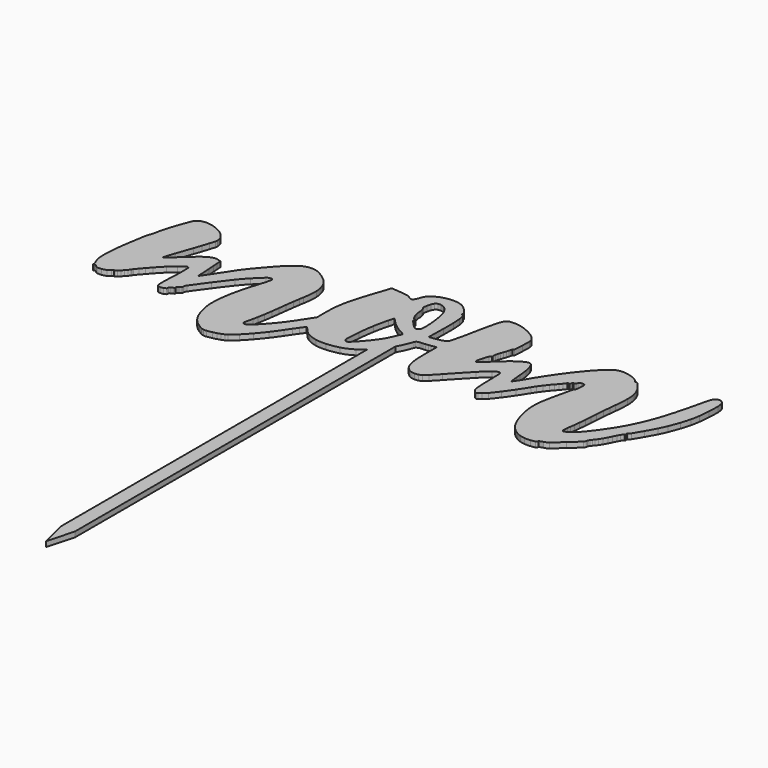
from build123d import *

# Parameters (mm, degrees)
F1_DEPTH = 1.5
F2_W     = 4
F2_H     = 115
F3_DEPTH = 1.5


# Not quite as in the source:
# - ends of sketch curves that miss each other by under 0.0002 mm in the source are joined


with BuildPart() as f1:
    # F0 (on Top) → F1 (new body)
    with BuildSketch(Plane.XY):
        with BuildLine():
            ThreePointArc((-4.1822559425, 22.5586507226), (-4.9915219103, 22.2917572117), (-5.7695987676, 21.9442806557))
            ThreePointArc((-5.7695987676, 21.9442806557), (-6.2638855218, 21.6755378797), (-6.742794415, 21.3802611645))
            ThreePointArc((-6.742794415, 21.3802611645), (-7.0841996448, 21.125395576), (-7.3917539608, 20.8305662103))
            ThreePointArc((-7.3917539608, 20.8305662103), (-7.6477142146, 20.5133884844), (-7.8596836812, 20.1652702398))
            ThreePointArc((-7.8596836812, 20.1652702398), (-8.0756822418, 19.7125223093), (-8.2587705459, 19.2454947615))
            ThreePointArc((-8.2587705459, 19.2454947615), (-8.4853451121, 18.6537844208), (-8.7444978395, 18.0756001689))
            ThreePointArc((-8.7444978395, 18.0756001689), (-8.9340338612, 17.8082033995), (-9.2009096557, 17.6179345962))
            ThreePointArc((-9.2009096557, 17.6179345962), (-9.4804778392, 17.5526269678), (-9.7609347332, 17.6140061624))
            ThreePointArc((-9.7609347332, 17.6140061624), (-10.1884309035, 17.8422128124), (-10.5897050006, 18.1138934121))
            ThreePointArc((-10.5897050006, 18.1138934121), (-10.9867832416, 18.3421223205), (-11.4282019209, 18.4642251951))
            ThreePointArc((-11.4282019209, 18.4642251951), (-12.5305443305, 18.6102904676), (-13.636129456, 18.7293508491))
            ThreePointArc((-13.636129456, 18.7293508491), (-14.7733093794, 18.8288693961), (-15.9118961479, 18.9107369284))
            ThreePointArc((-15.9118961479, 18.9107369284), (-16.1103487756, 18.8404745111), (-16.1965585813, 18.648411639))
            ThreePointArc((-16.1965585813, 18.648411639), (-16.200373914, 18.6073011501), (-16.210286377, 18.5672215402))
            ThreePointArc((-16.210286377, 18.5672215402), (-16.419979603, 17.9292142659), (-16.6298537231, 17.2912664743))
            ThreePointArc((-16.6298537231, 17.2912664743), (-16.8667329929, 16.574072426), (-17.1050936702, 15.8573693638))
            ThreePointArc((-17.1050936702, 15.8573693638), (-17.3865224907, 15.0158730838), (-17.6690280218, 14.1747376637))
            ThreePointArc((-17.6690280218, 14.1747376637), (-18.3536086298, 12.0776659538), (-18.9998070552, 9.9684509451))
            ThreePointArc((-18.9998070552, 9.9684509451), (-19.434349035, 8.3783522453), (-19.8004649353, 6.771118674))
            ThreePointArc((-19.8004649353, 6.771118674), (-20.0490192241, 5.3746056153), (-20.2234246645, 3.9669086683))
            ThreePointArc((-20.2234246645, 3.9669086683), (-20.3294158982, 2.5100215792), (-20.3647728593, 1.0497120123))
            Line((-20.3647728593, 1.0497120123), (-20.3647728593, -2.4233168496))
            Line((-20.3647728593, -2.4233168496), (-22.919139759, -6.3134028131))
            ThreePointArc((-22.919139759, -6.3134028131), (-23.9837763775, -7.8648103517), (-25.110819257, -9.3714924057))
            ThreePointArc((-25.110819257, -9.3714924057), (-26.2997155674, -10.8327814282), (-27.5470323246, -12.2445324531))
            ThreePointArc((-27.5470323246, -12.2445324531), (-28.6699490161, -13.4282570975), (-29.8280346413, -14.5775976193))
            ThreePointArc((-29.8280346413, -14.5775976193), (-30.3391428464, -14.9087464889), (-30.9370028544, -15.0247401796))
            ThreePointArc((-30.9370028544, -15.0247401796), (-31.1663651817, -14.9984768587), (-31.3838541049, -14.9210468419))
            ThreePointArc((-31.3838541049, -14.9210468419), (-31.5089949751, -14.808872531), (-31.5571193403, -14.6478527512))
            ThreePointArc((-31.5571193403, -14.6478527512), (-31.5428967438, -14.3333788672), (-31.4906101134, -14.0229562465))
            ThreePointArc((-31.4906101134, -14.0229562465), (-31.2411328819, -12.9594000391), (-30.985931045, -11.8972029212))
            ThreePointArc((-30.985931045, -11.8972029212), (-30.8380868978, -11.2453452123), (-30.7104532496, -10.5892308852))
            ThreePointArc((-30.7104532496, -10.5892308852), (-30.5374868635, -9.5932928505), (-30.3739315542, -8.5957661091))
            ThreePointArc((-30.3739315542, -8.5957661091), (-30.2012078519, -7.4762107698), (-30.0390624167, -6.3550745191))
            ThreePointArc((-30.0390624167, -6.3550745191), (-29.8922592615, -5.2641425918), (-29.7566894255, -4.1717578345))
            ThreePointArc((-29.7566894255, -4.1717578345), (-29.6251269486, -3.0895293391), (-29.4878411294, -2.0080119761))
            ThreePointArc((-29.4878411294, -2.0080119761), (-29.3435223079, -0.916672936), (-29.1935983974, 0.17391023))
            ThreePointArc((-29.1935983974, 0.17391023), (-29.0568759692, 1.1321864661), (-28.9152986168, 2.0897574667))
            ThreePointArc((-28.9152986168, 2.0897574667), (-28.8192464519, 2.6893466621), (-28.7117907934, 3.2869974804))
            ThreePointArc((-28.7117907934, 3.2869974804), (-28.4328255875, 5.2872447136), (-28.3503002579, 7.3051644583))
            ThreePointArc((-28.3503002579, 7.3051644583), (-28.5212434867, 8.8744231228), (-29.0021338886, 10.37793196))
            ThreePointArc((-29.0021338886, 10.37793196), (-29.7451965352, 11.6773360862), (-30.7525232215, 12.7845334956))
            ThreePointArc((-30.7525232215, 12.7845334956), (-32.16418877, 13.8757158075), (-33.7057215553, 14.7741339442))
            ThreePointArc((-33.7057215553, 14.7741339442), (-34.9524958644, 15.2120375761), (-36.2687880295, 15.3285737489))
            ThreePointArc((-36.2687880295, 15.3285737489), (-37.5645264585, 15.1148542043), (-38.764947663, 14.5823103026))
            ThreePointArc((-38.764947663, 14.5823103026), (-40.3221476085, 13.4878304003), (-41.7164387191, 12.1921799081))
            ThreePointArc((-41.7164387191, 12.1921799081), (-43.9120092144, 9.7823205671), (-46.0338372664, 7.3072857043))
            ThreePointArc((-46.0338372664, 7.3072857043), (-46.4456634194, 6.8082415191), (-46.8538054567, 6.3061798129))
            ThreePointArc((-46.8538054567, 6.3061798129), (-47.235224243, 5.8291917787), (-47.612454984, 5.3488847494))
            ThreePointArc((-47.612454984, 5.3488847494), (-47.9271786213, 4.9413426126), (-48.2387883176, 4.5314146198))
            ThreePointArc((-48.2387883176, 4.5314146198), (-48.3814207795, 4.3308497903), (-48.5126087033, 4.1226191562))
            ThreePointArc((-48.5126087033, 4.1226191562), (-48.6473158751, 3.9001325822), (-48.7865416946, 3.6804453742))
            ThreePointArc((-48.7865416946, 3.6804453742), (-49.1331745219, 3.1467861518), (-49.4808420237, 2.6138004196))
            ThreePointArc((-49.4808420237, 2.6138004196), (-49.8968100308, 1.9791749235), (-50.3143492141, 1.3455820469))
            ThreePointArc((-50.3143492141, 1.3455820469), (-50.7680770752, 0.6603827725), (-51.2231413323, -0.0239296847))
            Line((-51.2231413323, -0.0239296847), (-53.5166684536, -3.4655815887))
            Line((-53.5166684536, -3.4655815887), (-53.7783240639, 0.8672097846))
            ThreePointArc((-53.7783240639, 0.8672097846), (-53.8294707555, 1.6999810285), (-53.8823208533, 2.5326459042))
            ThreePointArc((-53.8823208533, 2.5326459042), (-53.9290447639, 3.2386970453), (-53.9781283051, 3.944588074))
            ThreePointArc((-53.9781283051, 3.944588074), (-54.0230894341, 4.5743024761), (-54.0682833336, 5.2040002153))
            ThreePointArc((-54.0682833336, 5.2040002153), (-54.0752279531, 5.2333667956), (-54.0910777713, 5.2590457477))
            ThreePointArc((-54.0910777713, 5.2590457477), (-54.1122644757, 5.2775060716), (-54.1377439385, 5.2893575669))
            ThreePointArc((-54.1377439385, 5.2893575669), (-54.2859965399, 5.3339698764), (-54.434460934, 5.3778722185))
            ThreePointArc((-54.434460934, 5.3778722185), (-54.6087752013, 5.4278455529), (-54.7836692699, 5.4757502762))
            ThreePointArc((-54.7836692699, 5.4757502762), (-54.9857744892, 5.5289837999), (-55.1882867028, 5.5806474337))
            ThreePointArc((-55.1882867028, 5.5806474337), (-55.7750569441, 5.6525847428), (-56.3615460507, 5.5783902643))
            ThreePointArc((-56.3615460507, 5.5783902643), (-57.0397471351, 5.3530815554), (-57.6792417151, 5.0340715138))
            ThreePointArc((-57.6792417151, 5.0340715138), (-58.5489239003, 4.4695325207), (-59.3681127786, 3.8339375469))
            ThreePointArc((-59.3681127786, 3.8339375469), (-60.6078625294, 2.7611061181), (-61.8227559636, 1.6602061928))
            ThreePointArc((-61.8227559636, 1.6602061928), (-62.4322452312, 1.0981496578), (-63.0447760209, 0.5394093375))
            ThreePointArc((-63.0447760209, 0.5394093375), (-63.5721918871, 0.0650609012), (-64.1036845799, -0.4047150597))
            ThreePointArc((-64.1036845799, -0.4047150597), (-64.5687800812, -0.81133911), (-65.0347655754, -1.2169429345))
            ThreePointArc((-65.0347655754, -1.2169429345), (-65.0929570576, -1.2515369423), (-65.1595758219, -1.2635759706))
            ThreePointArc((-65.1595758219, -1.2635759706), (-65.2465892772, -1.2202875127), (-65.264550455, -1.1247750628))
            ThreePointArc((-65.264550455, -1.1247750628), (-65.1010382295, -0.5630542496), (-64.9291088642, -0.0038523054))
            ThreePointArc((-64.9291088642, -0.0038523054), (-64.6191741236, 0.9558542093), (-64.2966272322, 1.9113957541))
            ThreePointArc((-64.2966272322, 1.9113957541), (-63.5118912001, 4.1817279915), (-62.7241409714, 6.4510161364))
            ThreePointArc((-62.7241409714, 6.4510161364), (-62.3584274565, 7.5153052648), (-62.0008194789, 8.5823452167))
            ThreePointArc((-62.0008194789, 8.5823452167), (-61.6896775555, 9.5395945184), (-61.3887147953, 10.5000927935))
            ThreePointArc((-61.3887147953, 10.5000927935), (-61.1430588832, 11.308414842), (-60.9027515407, 12.1183430759))
            ThreePointArc((-60.9027515407, 12.1183430759), (-60.8475182031, 12.3678683627), (-60.826260255, 12.6225479491))
            ThreePointArc((-60.826260255, 12.6225479491), (-60.8760261629, 13.2132637936), (-61.0422047693, 13.7823037851))
            ThreePointArc((-61.0422047693, 13.7823037851), (-61.3327877583, 14.3721380824), (-61.7067140299, 14.9129912493))
            ThreePointArc((-61.7067140299, 14.9129912493), (-62.2131221431, 15.4658692638), (-62.7850651647, 15.950641847))
            ThreePointArc((-62.7850651647, 15.950641847), (-63.4832237539, 16.4237718816), (-64.2206136701, 16.8330804933))
            ThreePointArc((-64.2206136701, 16.8330804933), (-65.1252901816, 17.2383089572), (-66.0602335864, 17.5677486859))
            ThreePointArc((-66.0602335864, 17.5677486859), (-66.9070821685, 17.7724206835), (-67.7724364315, 17.8734411577))
            ThreePointArc((-67.7724364315, 17.8734411577), (-68.5155243267, 17.8609951412), (-69.2490163874, 17.7413126029))
            ThreePointArc((-69.2490163874, 17.7413126029), (-69.853154693, 17.5236256148), (-70.3941183825, 17.1776067625))
            ThreePointArc((-70.3941183825, 17.1776067625), (-70.8092834506, 16.7433928091), (-71.1018494221, 16.2186938699))
            ThreePointArc((-71.1018494221, 16.2186938699), (-71.6814891859, 14.7304548726), (-72.231005615, 13.2308318357))
            ThreePointArc((-72.231005615, 13.2308318357), (-72.7813626503, 11.6050767122), (-73.2835471725, 9.9638018107))
            ThreePointArc((-73.2835471725, 9.9638018107), (-73.664727082, 8.5280649184), (-73.9804265564, 7.076523538))
            ThreePointArc((-73.9804265564, 7.076523538), (-74.0261796134, 6.8535167435), (-74.076771101, 6.6315575731))
            ThreePointArc((-74.076771101, 6.6315575731), (-74.135954279, 6.3934993523), (-74.1992682126, 6.1565062898))
            ThreePointArc((-74.1992682126, 6.1565062898), (-74.2617462221, 5.9380485217), (-74.328061585, 5.7207248687))
            ThreePointArc((-74.328061585, 5.7207248687), (-74.3814168207, 5.5633688503), (-74.4416203428, 5.4085036385))
            ThreePointArc((-74.4416203428, 5.4085036385), (-74.4994993237, 5.2601300671), (-74.5511683002, 5.1094814382))
            ThreePointArc((-74.5511683002, 5.1094814382), (-74.6108233058, 4.9162070008), (-74.6664979641, 4.7217486211))
            ThreePointArc((-74.6664979641, 4.7217486211), (-74.7202513052, 4.5183855512), (-74.7698584316, 4.3139715286))
            ThreePointArc((-74.7698584316, 4.3139715286), (-74.8092636056, 4.1320166537), (-74.8433256505, 3.9489862685))
            ThreePointArc((-74.8433256505, 3.9489862685), (-75.3714936754, 0.7359748324), (-75.8583007895, -2.4835628313))
            ThreePointArc((-75.8583007895, -2.4835628313), (-76.1231681958, -4.629163355), (-76.2985191984, -6.7839274669))
            ThreePointArc((-76.2985191984, -6.7839274669), (-76.3428147207, -8.2970233342), (-76.2929072344, -9.8099444977))
            ThreePointArc((-76.2929072344, -9.8099444977), (-76.1345866751, -10.8741643639), (-75.8013874655, -11.8972027673))
            ThreePointArc((-75.8013874655, -11.8972027673), (-75.6999104882, -12.1479333715), (-75.6054305509, -12.4013834739))
            ThreePointArc((-75.6054305509, -12.4013834739), (-75.5247349489, -12.6402342171), (-75.4522677026, -12.8817087512))
            ThreePointArc((-75.4522677026, -12.8817087512), (-75.398642255, -13.0842728713), (-75.3513736965, -13.2884139943))
            ThreePointArc((-75.3513736965, -13.2884139943), (-75.3408090463, -13.3902479231), (-75.3524233081, -13.4919674365))
            ThreePointArc((-75.3524233081, -13.4919674365), (-75.3578141372, -13.5473192244), (-75.3493302057, -13.6022819056))
            ThreePointArc((-75.3493302057, -13.6022819056), (-75.3274262122, -13.6398650775), (-75.2902116395, -13.6623896439))
            ThreePointArc((-75.2902116395, -13.6623896439), (-75.2345411787, -13.6700441916), (-75.1792530029, -13.6599936843))
            ThreePointArc((-75.1792530029, -13.6599936843), (-75.1035087165, -13.6286877996), (-75.0315710199, -13.589416625))
            ThreePointArc((-75.0315710199, -13.589416625), (-74.9487622667, -13.5495723993), (-74.8594618396, -13.5278862888))
            ThreePointArc((-74.8594618396, -13.5278862888), (-74.7657183984, -13.5246792034), (-74.6731732176, -13.5399601928))
            ThreePointArc((-74.6731732176, -13.5399601928), (-74.5832645797, -13.5736545995), (-74.5014379699, -13.6238869091))
            ThreePointArc((-74.5014379699, -13.6238869091), (-74.4296336563, -13.6893500971), (-74.3711213165, -13.7669232111))
            ThreePointArc((-74.3711213165, -13.7669232111), (-74.0943971868, -14.0492003461), (-73.7232801093, -14.1853206266))
            ThreePointArc((-73.7232801093, -14.1853206266), (-73.1081117024, -14.2256966538), (-72.4928310229, -14.1870696251))
            ThreePointArc((-72.4928310229, -14.1870696251), (-71.8377271814, -14.0622844651), (-71.2028465133, -13.8581792676))
            ThreePointArc((-71.2028465133, -13.8581792676), (-70.7333802299, -13.6070314156), (-70.3361908816, -13.252469085))
            ThreePointArc((-70.3361908816, -13.252469085), (-70.1864087009, -13.0866749815), (-70.0328775637, -12.9243463791))
            ThreePointArc((-70.0328775637, -12.9243463791), (-69.9437306254, -12.8430726196), (-69.8451341813, -12.7735647379))
            ThreePointArc((-69.8451341813, -12.7735647379), (-69.8105070702, -12.7730112819), (-69.7934259349, -12.8031374144))
            ThreePointArc((-69.7934259349, -12.8031374144), (-69.8028215767, -12.8733789518), (-69.827754287, -12.9397153005))
            ThreePointArc((-69.827754287, -12.9397153005), (-69.8245031219, -12.9853701203), (-69.7825618234, -13.0036965528))
            ThreePointArc((-69.7825618234, -13.0036965528), (-69.6947559153, -12.9801297562), (-69.6159866251, -12.9347350445))
            ThreePointArc((-69.6159866251, -12.9347350445), (-69.4087154408, -12.767215773), (-69.2106525463, -12.5889038654))
            ThreePointArc((-69.2106525463, -12.5889038654), (-68.9316613256, -12.3191357057), (-68.6575720048, -12.0443885362))
            ThreePointArc((-68.6575720048, -12.0443885362), (-68.3643476946, -11.7405929424), (-68.0757154403, -11.4324311665))
            ThreePointArc((-68.0757154403, -11.4324311665), (-67.8151289864, -11.1444754722), (-67.5601404874, -10.851551169))
            ThreePointArc((-67.5601404874, -10.851551169), (-67.3518605409, -10.6037065546), (-67.147453089, -10.3526585847))
            ThreePointArc((-67.147453089, -10.3526585847), (-67.0716457549, -10.2412100141), (-67.0141409908, -10.1193054142))
            ThreePointArc((-67.0141409908, -10.1193054142), (-66.9483485935, -9.9811894042), (-66.8608755299, -9.855677946))
            ThreePointArc((-66.8608755299, -9.855677946), (-66.4558544705, -9.3681557388), (-66.0483968957, -8.8826680599))
            ThreePointArc((-66.0483968957, -8.8826680599), (-65.5626572142, -8.3125097497), (-65.0713750069, -7.7471202124))
            ThreePointArc((-65.0713750069, -7.7471202124), (-64.5087102139, -7.1102408743), (-63.9417931494, -6.477143721))
            ThreePointArc((-63.9417931494, -6.477143721), (-62.8969404894, -5.3490949705), (-61.8220698579, -4.2496113755))
            ThreePointArc((-61.8220698579, -4.2496113755), (-60.9263888483, -3.4028181835), (-59.9880774003, -2.6035217377))
            ThreePointArc((-59.9880774003, -2.6035217377), (-59.262628442, -2.0479626884), (-58.5091525982, -1.5310524402))
            ThreePointArc((-58.5091525982, -1.5310524402), (-58.1616557398, -1.4262262904), (-57.8119768273, -1.5235258845))
            ThreePointArc((-57.8119768273, -1.5235258845), (-57.7137215941, -1.6246169813), (-57.6748883547, -1.7601363133))
            ThreePointArc((-57.6748883547, -1.7601363133), (-57.6538185631, -2.5029076798), (-57.6396808543, -3.2458433181))
            ThreePointArc((-57.6396808543, -3.2458433181), (-57.6360432054, -4.1307602045), (-57.6505451458, -5.0155657315))
            ThreePointArc((-57.6505451458, -5.0155657315), (-57.6846924586, -6.0447961381), (-57.7322697912, -7.07349321))
            ThreePointArc((-57.7322697912, -7.07349321), (-57.7944578959, -8.3689613454), (-57.8442692694, -9.6649643838))
            ThreePointArc((-57.8442692694, -9.6649643838), (-57.856867574, -10.4757670984), (-57.8401082345, -11.286494475))
            ThreePointArc((-57.8401082345, -11.286494475), (-57.807360429, -11.8159482663), (-57.7502999635, -12.3433360171))
            ThreePointArc((-57.7502999635, -12.3433360171), (-57.673204314, -12.5529847958), (-57.5136494411, -12.7093133269))
            ThreePointArc((-57.5136494411, -12.7093133269), (-57.2054591723, -12.8426456929), (-56.8719905685, -12.8821103557))
            ThreePointArc((-56.8719905685, -12.8821103557), (-56.4211425786, -12.8420036032), (-55.9785762085, -12.7470959978))
            ThreePointArc((-55.9785762085, -12.7470959978), (-55.6225780145, -12.6171325954), (-55.2909196385, -12.4337534234))
            ThreePointArc((-55.2909196385, -12.4337534234), (-55.1755300418, -12.2660820174), (-55.2095904797, -12.0654121401))
            ThreePointArc((-55.2095904797, -12.0654121401), (-55.2429992614, -11.9770427378), (-55.2408434003, -11.8825934375))
            ThreePointArc((-55.2408434003, -11.8825934375), (-55.2042535921, -11.7811978242), (-55.1425856263, -11.6927843572))
            ThreePointArc((-55.1425856263, -11.6927843572), (-55.0388849343, -11.5981176824), (-54.9198375465, -11.5236641951))
            ThreePointArc((-54.9198375465, -11.5236641951), (-54.7659971521, -11.4558390196), (-54.6058283114, -11.4047208545))
            ThreePointArc((-54.6058283114, -11.4047208545), (-54.4447093367, -11.3547072715), (-54.2887639942, -11.2903509784))
            ThreePointArc((-54.2887639942, -11.2903509784), (-54.167268058, -11.2214926632), (-54.058122806, -11.134371819))
            ThreePointArc((-54.058122806, -11.134371819), (-53.9924301765, -11.0560024408), (-53.9473415092, -10.9642184766))
            ThreePointArc((-53.9473415092, -10.9642184766), (-53.937987883, -10.8823035628), (-53.9647940919, -10.8043358161))
            ThreePointArc((-53.9647940919, -10.8043358161), (-53.9964262926, -10.7265964996), (-54.000804246, -10.6427822877))
            ThreePointArc((-54.000804246, -10.6427822877), (-53.978910261, -10.5513457426), (-53.935896193, -10.4677408564))
            ThreePointArc((-53.935896193, -10.4677408564), (-53.8631232474, -10.3789790757), (-53.7754141586, -10.30494073))
            ThreePointArc((-53.7754141586, -10.30494073), (-53.6630098407, -10.2362111231), (-53.5430990436, -10.1816227544))
            ThreePointArc((-53.5430990436, -10.1816227544), (-53.4154851319, -10.1256275996), (-53.2937010792, -10.0578824381))
            ThreePointArc((-53.2937010792, -10.0578824381), (-53.1838223253, -9.9814396197), (-53.0826675643, -9.8937779729))
            ThreePointArc((-53.0826675643, -9.8937779729), (-53.0050697908, -9.8093331136), (-52.9382242426, -9.7161450243))
            ThreePointArc((-52.9382242426, -9.7161450243), (-52.9031619045, -9.637914576), (-52.8911609896, -9.5530302369))
            ThreePointArc((-52.8911609896, -9.5530302369), (-52.8055751283, -9.0065852313), (-52.5570144162, -8.5124752676))
            ThreePointArc((-52.5570144162, -8.5124752676), (-50.9049322696, -6.2203896441), (-49.2387076685, -3.9385641684))
            ThreePointArc((-49.2387076685, -3.9385641684), (-47.620417887, -1.7722741308), (-45.9685796397, 0.368544584))
            ThreePointArc((-45.9685796397, 0.368544584), (-44.8534491069, 1.7140619809), (-43.6671281303, 2.9972516342))
            ThreePointArc((-43.6671281303, 2.9972516342), (-42.4301332189, 4.2308010058), (-41.1602271105, 5.4304421727))
            ThreePointArc((-41.1602271105, 5.4304421727), (-40.6342141081, 5.7522390789), (-40.0254736735, 5.8506163559))
            ThreePointArc((-40.0254736735, 5.8506163559), (-39.6468333598, 5.661340297), (-39.5427213099, 5.2510300767))
            ThreePointArc((-39.5427213099, 5.2510300767), (-39.8013508117, 4.0542865399), (-40.1358962279, 2.8765074091))
            ThreePointArc((-40.1358962279, 2.8765074091), (-41.025635013, -0.0511910088), (-41.8349245611, -3.0021406109))
            ThreePointArc((-41.8349245611, -3.0021406109), (-42.3726246239, -5.3408386427), (-42.7786081902, -7.7059617258))
            ThreePointArc((-42.7786081902, -7.7059617258), (-42.985017337, -9.6396450101), (-43.0531009585, -11.5831213836))
            ThreePointArc((-43.0531009585, -11.5831213836), (-42.9576359866, -13.2428668027), (-42.6746090087, -14.8810866201))
            ThreePointArc((-42.6746090087, -14.8810866201), (-42.3511388295, -16.1104284713), (-41.9559710395, -17.3186324001))
            ThreePointArc((-41.9559710395, -17.3186324001), (-41.5479934206, -18.2935342997), (-41.0431893663, -19.2220020331))
            ThreePointArc((-41.0431893663, -19.2220020331), (-40.4997867922, -20.0043819358), (-39.8691379588, -20.7183053858))
            ThreePointArc((-39.8691379588, -20.7183053858), (-39.1527041487, -21.3630475184), (-38.3684380392, -21.9233121883))
            ThreePointArc((-38.3684380392, -21.9233121883), (-37.7803696665, -22.2807581428), (-37.1798687644, -22.6168990168))
            ThreePointArc((-37.1798687644, -22.6168990168), (-36.8187592337, -22.7726530636), (-36.4364715582, -22.8649328236))
            ThreePointArc((-36.4364715582, -22.8649328236), (-36.0255703165, -22.8960166594), (-35.6147111703, -22.8643813839))
            ThreePointArc((-35.6147111703, -22.8643813839), (-34.8322051067, -22.73353173), (-34.05326431, -22.5829043212))
            ThreePointArc((-34.05326431, -22.5829043212), (-33.5450667482, -22.4683826133), (-33.0413101397, -22.3356827592))
            ThreePointArc((-33.0413101397, -22.3356827592), (-32.5382415862, -22.1838969881), (-32.0407933742, -22.0145979308))
            ThreePointArc((-32.0407933742, -22.0145979308), (-31.6088795425, -21.8504218929), (-31.1830483815, -21.6710587133))
            ThreePointArc((-31.1830483815, -21.6710587133), (-30.9156435461, -21.5330041438), (-30.6667650025, -21.3638182089))
            ThreePointArc((-30.6667650025, -21.3638182089), (-29.6790688612, -20.5493797605), (-28.7459929373, -19.6728964566))
            ThreePointArc((-28.7459929373, -19.6728964566), (-27.6334299799, -18.520275589), (-26.5598745739, -17.3312381615))
            ThreePointArc((-26.5598745739, -17.3312381615), (-25.4284265627, -15.9933166985), (-24.3397287735, -14.620383499))
            ThreePointArc((-24.3397287735, -14.620383499), (-23.2970435644, -13.2164689104), (-22.2994122978, -11.7801888303))
            ThreePointArc((-22.2994122978, -11.7801888303), (-21.7461323637, -10.9615839169), (-21.1877421009, -10.1464563169))
            ThreePointArc((-21.1877421009, -10.1464563169), (-20.7064388551, -9.4560230246), (-20.2181990799, -8.7704773517))
            ThreePointArc((-20.2181990799, -8.7704773517), (-19.7895503223, -8.1765157547), (-19.3594479355, -7.5836059198))
            ThreePointArc((-19.3594479355, -7.5836059198), (-19.3034623423, -7.5358243614), (-19.2318904369, -7.5186506111))
            ThreePointArc((-19.2318904369, -7.5186506111), (-19.1686419514, -7.5305800964), (-19.1140845066, -7.5647293093))
            ThreePointArc((-19.1140845066, -7.5647293093), (-18.9770961812, -7.6943381598), (-18.8432663523, -7.8272058875))
            ThreePointArc((-18.8432663523, -7.8272058875), (-18.6841706893, -7.9943686056), (-18.5306061244, -8.1666263419))
            ThreePointArc((-18.5306061244, -8.1666263419), (-18.3625456012, -8.3659621524), (-18.199040705, -8.5690514311))
            ThreePointArc((-18.199040705, -8.5690514311), (-17.3531301887, -9.4416557191), (-16.3461412481, -10.12207919))
            ThreePointArc((-16.3461412481, -10.12207919), (-15.1159644234, -10.6628346337), (-13.8175853913, -11.0091919713))
            ThreePointArc((-13.8175853913, -11.0091919713), (-12.2858853212, -11.1921895086), (-10.7433888506, -11.1749306796))
            ThreePointArc((-10.7433888506, -11.1749306796), (-9.0034596895, -10.9638456428), (-7.2891719049, -10.5989788562))
            ThreePointArc((-7.2891719049, -10.5989788562), (-5.5072879501, -9.9724728868), (-3.8550637645, -9.0571721758))
            ThreePointArc((-3.8550637645, -9.0571721758), (-2.1773976949, -7.7809088725), (-0.6661841912, -6.3113357406))
            ThreePointArc((-0.6661841912, -6.3113357406), (0.780118398, -4.5348463442), (2.0206413229, -2.6090211129))
            ThreePointArc((2.0206413229, -2.6090211129), (3.101013261, -0.4720664298), (3.9687420637, 1.7597100373))
            ThreePointArc((3.9687420637, 1.7597100373), (4.0429607856, 1.9222699293), (4.1497565079, 2.0655487572))
            ThreePointArc((4.1497565079, 2.0655487572), (4.2918637926, 2.1949479823), (4.4539218623, 2.2982717748))
            ThreePointArc((4.4539218623, 2.2982717748), (4.6559590459, 2.3860996721), (4.8685089146, 2.444024833))
            ThreePointArc((4.8685089146, 2.444024833), (5.1191629671, 2.4810197731), (5.3721967094, 2.4940583415))
            ThreePointArc((5.3721967094, 2.4940583415), (5.6474109783, 2.4993711533), (5.9223326228, 2.513126545))
            ThreePointArc((5.9223326228, 2.513126545), (6.2759538804, 2.5388542458), (6.6291626887, 2.5697321278))
            ThreePointArc((6.6291626887, 2.5697321278), (6.9984444577, 2.6074183955), (7.3671439486, 2.6504296454))
            ThreePointArc((7.3671439486, 2.6504296454), (7.6953045038, 2.6945009672), (8.0225027057, 2.7452253932))
            Line((8.0225027057, 2.7452253932), (9.512956874, 2.9918030159))
            Line((9.512956874, 2.9918030159), (9.489490753, -1.1166601135))
            ThreePointArc((9.489490753, -1.1166601135), (9.5312740917, -3.2067309573), (9.6803820608, -5.2918949357))
            ThreePointArc((9.6803820608, -5.2918949357), (9.9288893063, -6.6590144491), (10.3991588685, -7.9665380884))
            ThreePointArc((10.3991588685, -7.9665380884), (10.9353106418, -8.8055932953), (11.6832726288, -9.4628795794))
            ThreePointArc((11.6832726288, -9.4628795794), (12.5765507142, -9.8782528649), (13.551330224, -10.0206804672))
            ThreePointArc((13.551330224, -10.0206804672), (14.0908782717, -9.9864098255), (14.6217540504, -9.8841480039))
            ThreePointArc((14.6217540504, -9.8841480039), (15.0692994731, -9.7226182531), (15.4794268286, -9.4814040321))
            ThreePointArc((15.4794268286, -9.4814040321), (16.0162580118, -9.0571422232), (16.5132514964, -8.5868409476))
            ThreePointArc((16.5132514964, -8.5868409476), (17.5599755317, -7.4925098038), (18.5950103109, -6.387116271))
            ThreePointArc((18.5950103109, -6.387116271), (21.1766435374, -3.6230930989), (23.7806788264, -0.8801650253))
            ThreePointArc((23.7806788264, -0.8801650253), (25.0803561969, 0.4005733241), (26.4526707118, 1.6031559035))
            ThreePointArc((26.4526707118, 1.6031559035), (27.0922293683, 2.0133090023), (27.8109979968, 2.2595457583))
            ThreePointArc((27.8109979968, 2.2595457583), (28.2507574872, 2.159610569), (28.4592161085, 1.7597101107))
            ThreePointArc((28.4592161085, 1.7597101107), (28.4692596352, 1.5208514025), (28.4768725053, 1.2819028765))
            ThreePointArc((28.4768725053, 1.2819028765), (28.4939603313, 0.6342572533), (28.5105505023, -0.0134013091))
            ThreePointArc((28.5105505023, -0.0134013091), (28.5296330893, -0.7859654794), (28.5478966907, -1.5585494446))
            ThreePointArc((28.5478966907, -1.5585494446), (28.5671175763, -2.405090089), (28.5856563176, -3.2516459466))
            ThreePointArc((28.5856563176, -3.2516459466), (28.6169098518, -4.3551611664), (28.6632158116, -5.4581472845))
            ThreePointArc((28.6632158116, -5.4581472845), (28.7145806605, -6.1315653674), (28.8026823915, -6.8011684907))
            ThreePointArc((28.8026823915, -6.8011684907), (28.8942746689, -7.2434743103), (29.0261349776, -7.6754887276))
            ThreePointArc((29.0261349776, -7.6754887276), (29.1722350636, -7.9756000796), (29.3807156249, -8.236268275))
            ThreePointArc((29.3807156249, -8.236268275), (29.5964786231, -8.4357316695), (29.8272129846, -8.6176683828))
            ThreePointArc((29.8272129846, -8.6176683828), (29.9805902517, -8.6919159083), (30.1502157997, -8.7081781892))
            ThreePointArc((30.1502157997, -8.7081781892), (30.344043037, -8.6676523343), (30.5219808533, -8.5807645481))
            ThreePointArc((30.5219808533, -8.5807645481), (30.882288134, -8.3376876919), (31.2350483829, -8.0837823983))
            ThreePointArc((31.2350483829, -8.0837823983), (31.824369437, -7.5860863968), (32.3473243525, -7.0190601609))
            ThreePointArc((32.3473243525, -7.0190601609), (33.2476306791, -5.8866672621), (34.1227586607, -4.7347053781))
            ThreePointArc((34.1227586607, -4.7347053781), (35.124039662, -3.3523285847), (36.0924561327, -1.9467330607))
            ThreePointArc((36.0924561327, -1.9467330607), (37.0697547841, -0.4586636714), (38.015923698, 1.0493905546))
            ThreePointArc((38.015923698, 1.0493905546), (38.3518642472, 1.5801537477), (38.7028940485, 2.1010603574))
            ThreePointArc((38.7028940485, 2.1010603574), (39.1291275513, 2.7028892508), (39.5660063972, 3.2970356044))
            ThreePointArc((39.5660063972, 3.2970356044), (40.0082629291, 3.8765586045), (40.4607950996, 4.448093717))
            ThreePointArc((40.4607950996, 4.448093717), (40.844798252, 4.9090843036), (41.2432648985, 5.3576320424))
            ThreePointArc((41.2432648985, 5.3576320424), (41.5851348707, 5.7363994216), (41.9209004543, 6.1205885391))
            ThreePointArc((41.9209004543, 6.1205885391), (42.211029315, 6.4659643816), (42.4930970393, 6.8179544825))
            ThreePointArc((42.4930970393, 6.8179544825), (42.7215863159, 7.114423429), (42.9456715876, 7.4142349964))
            ThreePointArc((42.9456715876, 7.4142349964), (42.9969004516, 7.5128428476), (43.0155362051, 7.6223901518))
            ThreePointArc((43.0155362051, 7.6223901518), (43.0251743045, 7.6785512227), (43.0516651153, 7.7290011665))
            ThreePointArc((43.0516651153, 7.7290011665), (43.0911568068, 7.765392631), (43.1411722553, 7.7849473267))
            ThreePointArc((43.1411722553, 7.7849473267), (43.2095847052, 7.7891528451), (43.2769014286, 7.7762530513))
            ThreePointArc((43.2769014286, 7.7762530513), (43.3591638817, 7.7439279933), (43.4369884794, 7.7020310244))
            ThreePointArc((43.4369884794, 7.7020310244), (43.5129791306, 7.669172854), (43.5952014102, 7.6594911477))
            ThreePointArc((43.5952014102, 7.6594911477), (43.6689751089, 7.6757971942), (43.7314982919, 7.7182153395))
            ThreePointArc((43.7314982919, 7.7182153395), (43.7883356364, 7.7926435542), (43.8235723487, 7.8794099626))
            ThreePointArc((43.8235723487, 7.8794099626), (43.846357782, 7.9982613224), (43.853993449, 8.11903599))
            ThreePointArc((43.853993449, 8.11903599), (43.860750077, 8.2407770416), (43.8809369681, 8.3610227281))
            ThreePointArc((43.8809369681, 8.3610227281), (43.9122967737, 8.4493650521), (43.9636526974, 8.5277893835))
            ThreePointArc((43.9636526974, 8.5277893835), (44.0184996144, 8.5725231255), (44.0859195414, 8.5940599733))
            ThreePointArc((44.0859195414, 8.5940599733), (44.1592540039, 8.5906020528), (44.227302493, 8.563046519))
            ThreePointArc((44.227302493, 8.563046519), (44.3046897672, 8.5308526648), (44.3882673072, 8.5245262816))
            ThreePointArc((44.3882673072, 8.5245262816), (44.4783078954, 8.543275795), (44.5611909281, 8.5831412747))
            ThreePointArc((44.5611909281, 8.5831412747), (44.6480269664, 8.65115911), (44.7205143657, 8.7343005568))
            ThreePointArc((44.7205143657, 8.7343005568), (44.7872043737, 8.8410510944), (44.8397222007, 8.955441265))
            ThreePointArc((44.8397222007, 8.955441265), (44.9041820547, 9.0825220345), (44.9932755812, 9.1937287689))
            ThreePointArc((44.9932755812, 9.1937287689), (45.1167884794, 9.3033127422), (45.2537664321, 9.3955143001))
            ThreePointArc((45.2537664321, 9.3955143001), (45.4108469203, 9.473923384), (45.5765171971, 9.5320234226))
            ThreePointArc((45.5765171971, 9.5320234226), (45.7433904576, 9.5668660799), (45.9134613452, 9.5785534061))
            ThreePointArc((45.9134613452, 9.5785534061), (46.1301303931, 9.5599418238), (46.3404515124, 9.504652638))
            ThreePointArc((46.3404515124, 9.504652638), (46.4802101427, 9.4210873436), (46.5774055702, 9.2904401577))
            ThreePointArc((46.5774055702, 9.2904401577), (46.6497411129, 9.0830956188), (46.6760384006, 8.865075824))
            ThreePointArc((46.6760384006, 8.865075824), (46.6737045744, 8.4397555193), (46.6563078263, 8.0147847418))
            ThreePointArc((46.6563078263, 8.0147847418), (46.6337783198, 7.7073264378), (46.6023310556, 7.4006519257))
            ThreePointArc((46.6023310556, 7.4006519257), (46.5644129946, 7.1240431875), (46.5157243685, 6.8491257653))
            ThreePointArc((46.5157243685, 6.8491257653), (46.4678028856, 6.6262150774), (46.4123554205, 6.4050562554))
            ThreePointArc((46.4123554205, 6.4050562554), (46.3723559832, 6.315410401), (46.306611178, 6.2425135442))
            ThreePointArc((46.306611178, 6.2425135442), (46.1179309146, 6.0300746205), (46.0081185178, 5.7680215759))
            ThreePointArc((46.0081185178, 5.7680215759), (45.5958517596, 4.0074060445), (45.1909550712, 2.2450809889))
            ThreePointArc((45.1909550712, 2.2450809889), (44.8186008855, 0.5565252698), (44.4688955631, -1.1368660738))
            ThreePointArc((44.4688955631, -1.1368660738), (44.2508355318, -2.3434245024), (44.0767173661, -3.5571033252))
            ThreePointArc((44.0767173661, -3.5571033252), (43.9568623474, -5.3612491253), (44.0466276671, -7.1671421024))
            ThreePointArc((44.0466276671, -7.1671421024), (44.3464804573, -9.1352910314), (44.8162953961, -11.0699217004))
            ThreePointArc((44.8162953961, -11.0699217004), (45.4252769616, -12.868264555), (46.192593117, -14.6049630041))
            ThreePointArc((46.192593117, -14.6049630041), (46.9872445976, -15.9163716112), (47.9899713418, -17.0764589326))
            ThreePointArc((47.9899713418, -17.0764589326), (48.2845264269, -17.3443360137), (48.5976063222, -17.5903071722))
            ThreePointArc((48.5976063222, -17.5903071722), (48.9786013838, -17.8549041382), (49.3712982873, -18.1018007347))
            ThreePointArc((49.3712982873, -18.1018007347), (49.7713137011, -18.3284200401), (50.1813067407, -18.5364449076))
            ThreePointArc((50.1813067407, -18.5364449076), (50.5347061511, -18.6890837531), (50.8988930408, -18.813814152))
            ThreePointArc((50.8988930408, -18.813814152), (51.5671485515, -18.9727164233), (52.249247296, -19.0536896794))
            ThreePointArc((52.249247296, -19.0536896794), (53.0411729461, -19.0717371286), (53.8322056975, -19.0300342333))
            ThreePointArc((53.8322056975, -19.0300342333), (54.5186325178, -18.9441821841), (55.1976326329, -18.8118522884))
            ThreePointArc((55.1976326329, -18.8118522884), (55.4368640095, -18.6610062478), (55.5301327778, -18.3940098633))
            ThreePointArc((55.5301327778, -18.3940098633), (55.5495968182, -18.3108056363), (55.6039494215, -18.2448694037))
            ThreePointArc((55.6039494215, -18.2448694037), (55.7317548897, -18.1561627418), (55.8669948597, -18.0792650131))
            ThreePointArc((55.8669948597, -18.0792650131), (56.0493011005, -17.9950375299), (56.2376655624, -17.9254051846))
            ThreePointArc((56.2376655624, -17.9254051846), (56.4556902739, -17.8609249585), (56.676896482, -17.8083865193))
            ThreePointArc((56.676896482, -17.8083865193), (57.290048042, -17.5984311027), (57.8329751069, -17.2445013385))
            ThreePointArc((57.8329751069, -17.2445013385), (59.265399127, -16.0142080276), (60.6778838304, -14.7610730943))
            ThreePointArc((60.6778838304, -14.7610730943), (62.1062858033, -13.4577775901), (63.5191700656, -12.1376755337))
            ThreePointArc((63.5191700656, -12.1376755337), (63.7787347989, -11.766346072), (63.8702322984, -11.3226258811))
            ThreePointArc((63.8702322984, -11.3226258811), (63.8839439252, -11.2217947209), (63.9240829882, -11.128286501))
            ThreePointArc((63.9240829882, -11.128286501), (64.049353121, -10.926228771), (64.1803677558, -10.7278475816))
            ThreePointArc((64.1803677558, -10.7278475816), (64.347079519, -10.4917955687), (64.5216724596, -10.2615116765))
            ThreePointArc((64.5216724596, -10.2615116765), (64.7207161937, -10.0145629444), (64.9260123831, -9.7727870955))
            ThreePointArc((64.9260123831, -9.7727870955), (65.1765917756, -9.4655249997), (65.4065944877, -9.1425717756))
            ThreePointArc((65.4065944877, -9.1425717756), (65.7045461631, -8.681348528), (65.9907266425, -8.2127305346))
            ThreePointArc((65.9907266425, -8.2127305346), (66.2892362047, -7.6951177968), (66.5747459924, -7.1702225112))
            ThreePointArc((66.5747459924, -7.1702225112), (66.8289631129, -6.6705254848), (67.0679849654, -6.1633844611))
            ThreePointArc((67.0679849654, -6.1633844611), (67.2843221112, -5.7012082861), (67.5120940205, -5.2445590394))
            ThreePointArc((67.5120940205, -5.2445590394), (67.722825561, -4.8531618815), (67.9481043082, -4.469953054))
            ThreePointArc((67.9481043082, -4.469953054), (68.1397081049, -4.167178215), (68.3396979053, -3.869875849))
            ThreePointArc((68.3396979053, -3.869875849), (68.426448711, -3.7932502123), (68.5388452849, -3.7656058268))
            ThreePointArc((68.5388452849, -3.7656058268), (68.6044681861, -3.7579620356), (68.6665772831, -3.7354397626))
            ThreePointArc((68.6665772831, -3.7354397626), (68.7115299637, -3.7014436462), (68.7412764282, -3.6535727868))
            ThreePointArc((68.7412764282, -3.6535727868), (68.7548422747, -3.5924229027), (68.7492275609, -3.5300384823))
            ThreePointArc((68.7492275609, -3.5300384823), (68.7241724031, -3.4547445408), (68.6878015372, -3.3842172521))
            ThreePointArc((68.6878015372, -3.3842172521), (68.6490083815, -3.3086812116), (68.6226051159, -3.227975122))
            ThreePointArc((68.6226051159, -3.227975122), (68.6122843607, -3.151115113), (68.6179892523, -3.0737754208))
            ThreePointArc((68.6179892523, -3.0737754208), (68.6384802434, -3.0065493269), (68.6742035781, -2.9460260264))
            ThreePointArc((68.6742035781, -2.9460260264), (68.7222733519, -2.8975441535), (68.7811392943, -2.8629608848))
            ThreePointArc((68.7811392943, -2.8629608848), (69.1292771623, -2.645946491), (69.3943110903, -2.3328134946))
            ThreePointArc((69.3943110903, -2.3328134946), (70.1978899599, -0.995842331), (70.9861269272, 0.3502309881))
            ThreePointArc((70.9861269272, 0.3502309881), (71.7641731636, 1.7327100523), (72.5104368534, 3.1326010462))
            ThreePointArc((72.5104368534, 3.1326010462), (73.0619622657, 4.2585372049), (73.5614515174, 5.4085037246))
            ThreePointArc((73.5614515174, 5.4085037246), (74.1680794068, 6.9577497079), (74.7320598466, 8.5230249527))
            ThreePointArc((74.7320598466, 8.5230249527), (75.1464259985, 9.8269558513), (75.4965727481, 11.1495791388))
            ThreePointArc((75.4965727481, 11.1495791388), (75.7683208052, 12.4342910774), (75.9731834469, 13.7313504563))
            ThreePointArc((75.9731834469, 13.7313504563), (76.1408864175, 15.2101650715), (76.2557647003, 16.6940181472))
            ThreePointArc((76.2557647003, 16.6940181472), (76.3225950862, 18.2101689013), (76.3427471023, 19.7276580427))
            ThreePointArc((76.3427471023, 19.7276580427), (76.2750012132, 20.5691956002), (76.0769671895, 21.3899010737))
            ThreePointArc((76.0769671895, 21.3899010737), (75.8275857388, 21.8536117701), (75.4319250346, 22.200989627))
            ThreePointArc((75.4319250346, 22.200989627), (74.9286471696, 22.4004787128), (74.3878976108, 22.4264483489))
            ThreePointArc((74.3878976108, 22.4264483489), (74.0322792562, 22.3320326331), (73.7176668752, 22.1412506176))
            ThreePointArc((73.7176668752, 22.1412506176), (73.4500498339, 21.860129654), (73.2583313449, 21.5226509024))
            ThreePointArc((73.2583313449, 21.5226509024), (73.018196392, 20.876001781), (72.8291422801, 20.2126177095))
            ThreePointArc((72.8291422801, 20.2126177095), (72.404081372, 18.4414363322), (71.9900771171, 16.667637944))
            ThreePointArc((71.9900771171, 16.667637944), (71.015709787, 12.7537776104), (69.9025311659, 8.8771131008))
            ThreePointArc((69.9025311659, 8.8771131008), (68.8309806693, 5.7420333594), (67.561708613, 2.6816585686))
            ThreePointArc((67.561708613, 2.6816585686), (66.1963402676, -0.0715447728), (64.6400350137, -2.7215020025))
            ThreePointArc((64.6400350137, -2.7215020025), (62.7963510757, -5.4443881522), (60.7987277454, -8.056433417))
            ThreePointArc((60.7987277454, -8.056433417), (60.1860957259, -8.7656054686), (59.5310279116, -9.4357764709))
            ThreePointArc((59.5310279116, -9.4357764709), (58.9011893003, -9.9920475259), (58.2263133612, -10.4927236716))
            ThreePointArc((58.2263133612, -10.4927236716), (57.6958405036, -10.8129518785), (57.1346815262, -11.0757220432))
            ThreePointArc((57.1346815262, -11.0757220432), (56.8362408306, -11.0860844979), (56.6015426121, -10.9014469784))
            ThreePointArc((56.6015426121, -10.9014469784), (56.5484046992, -10.7800604769), (56.5311315724, -10.6486832894))
            ThreePointArc((56.5311315724, -10.6486832894), (56.538765521, -10.3166077053), (56.5548723368, -9.9848351286))
            ThreePointArc((56.5548723368, -9.9848351286), (56.5859711404, -9.5820736099), (56.6297697198, -9.1804946495))
            ThreePointArc((56.6297697198, -9.1804946495), (56.690394284, -8.7378262474), (56.7613424072, -8.2966947311))
            ThreePointArc((56.7613424072, -8.2966947311), (56.8519815762, -7.7272106675), (56.9274290921, -7.1555156138))
            ThreePointArc((56.9274290921, -7.1555156138), (57.0221075946, -6.3239028629), (57.1092314463, -5.4914647452))
            ThreePointArc((57.1092314463, -5.4914647452), (57.1971578129, -4.5709548165), (57.2767779909, -3.6496892737))
            ThreePointArc((57.2767779909, -3.6496892737), (57.3442400594, -2.7697126127), (57.4025695364, -1.8890834457))
            ThreePointArc((57.4025695364, -1.8890834457), (57.463379572, -0.9546447038), (57.5317247118, -0.0207268462))
            ThreePointArc((57.5317247118, -0.0207268462), (57.6185373631, 1.0670339194), (57.7109116998, 2.1543365001))
            ThreePointArc((57.7109116998, 2.1543365001), (57.807095394, 3.2216097525), (57.9087595045, 4.2883749132))
            ThreePointArc((57.9087595045, 4.2883749132), (57.9977081475, 5.1545970778), (58.0948747198, 6.0199359458))
            ThreePointArc((58.0948747198, 6.0199359458), (58.274353575, 7.974011843), (58.3560514311, 9.9346114336))
            ThreePointArc((58.3560514311, 9.9346114336), (58.2902339093, 11.3629758204), (58.046232907, 12.7718832952))
            ThreePointArc((58.046232907, 12.7718832952), (57.6657457047, 13.9495830271), (57.1062668993, 15.0535443518))
            ThreePointArc((57.1062668993, 15.0535443518), (56.3323364155, 16.1682941236), (55.4315153045, 17.1832605149))
            ThreePointArc((55.4315153045, 17.1832605149), (55.2926632801, 17.3165408867), (55.1484723369, 17.4440262353))
            ThreePointArc((55.1484723369, 17.4440262353), (55.0332421127, 17.5329242115), (54.9102687883, 17.6107600612))
            ThreePointArc((54.9102687883, 17.6107600612), (54.8348550703, 17.6442479556), (54.7542920975, 17.6620880844))
            ThreePointArc((54.7542920975, 17.6620880844), (54.7095669594, 17.6482947784), (54.6897375904, 17.6058991873))
            ThreePointArc((54.6897375904, 17.6058991873), (54.6815739811, 17.5633009457), (54.6597518256, 17.5258169968))
            ThreePointArc((54.6597518256, 17.5258169968), (54.6303139519, 17.506717243), (54.5952318099, 17.5075122977))
            ThreePointArc((54.5952318099, 17.5075122977), (54.5416446861, 17.53281619), (54.4955648867, 17.5700790777))
            ThreePointArc((54.4955648867, 17.5700790777), (54.4338615734, 17.6380722954), (54.3769836286, 17.7101505356))
            ThreePointArc((54.3769836286, 17.7101505356), (54.0315536407, 18.0926482282), (53.6164733286, 18.398155535))
            ThreePointArc((53.6164733286, 18.398155535), (52.9980087038, 18.7299896613), (52.3543596631, 19.009861553))
            ThreePointArc((52.3543596631, 19.009861553), (51.6364531262, 19.2550199627), (50.9012737541, 19.4421128437))
            ThreePointArc((50.9012737541, 19.4421128437), (50.2167579485, 19.5504335146), (49.524672729, 19.5866728308))
            ThreePointArc((49.524672729, 19.5866728308), (48.9808469668, 19.56953903), (48.4391783319, 19.5182056425))
            ThreePointArc((48.4391783319, 19.5182056425), (48.0308914207, 19.437549348), (47.6375959824, 19.3014525887))
            ThreePointArc((47.6375959824, 19.3014525887), (47.2377523049, 19.101806212), (46.8651260121, 18.8550608241))
            ThreePointArc((46.8651260121, 18.8550608241), (46.3484860388, 18.4492001389), (45.848574351, 18.02290438))
            ThreePointArc((45.848574351, 18.02290438), (44.5550300861, 16.7985625764), (43.3417532194, 15.4946343412))
            ThreePointArc((43.3417532194, 15.4946343412), (41.9112162335, 13.7998847716), (40.5377418469, 12.0585691001))
            ThreePointArc((40.5377418469, 12.0585691001), (39.0617131773, 10.0592537042), (37.6475157055, 8.0157351198))
            ThreePointArc((37.6475157055, 8.0157351198), (36.2264699073, 5.8315553565), (34.8638733778, 3.6104423283))
            ThreePointArc((34.8638733778, 3.6104423283), (34.4901495948, 2.9888536443), (34.1110585436, 2.3705236917))
            ThreePointArc((34.1110585436, 2.3705236917), (33.7878160414, 1.8568470947), (33.4570586109, 1.3479768891))
            ThreePointArc((33.4570586109, 1.3479768891), (33.1721371758, 0.9186887541), (32.8852971802, 0.490680175))
            ThreePointArc((32.8852971802, 0.490680175), (32.8435870288, 0.4660412619), (32.7981731574, 0.4829050383))
            ThreePointArc((32.7981731574, 0.4829050383), (32.7601754626, 0.5375197984), (32.7416468392, 0.6014203927))
            ThreePointArc((32.7416468392, 0.6014203927), (32.6825884732, 1.0998652891), (32.6249897504, 1.5984809651))
            ThreePointArc((32.6249897504, 1.5984809651), (32.5620342084, 2.175328164), (32.5046620142, 2.7527574006))
            ThreePointArc((32.5046620142, 2.7527574006), (32.4432229077, 3.4251956621), (32.3859270405, 4.0979996176))
            ThreePointArc((32.3859270405, 4.0979996176), (32.2642109208, 5.3418378083), (32.1035797041, 6.5812513282))
            ThreePointArc((32.1035797041, 6.5812513282), (31.9379327799, 7.464143022), (31.7006871447, 8.3305442952))
            ThreePointArc((31.7006871447, 8.3305442952), (31.476801739, 8.9088663842), (31.1840070289, 9.4555402952))
            ThreePointArc((31.1840070289, 9.4555402952), (30.9057572942, 9.7521035605), (30.5337690268, 9.916412396))
            ThreePointArc((30.5337690268, 9.916412396), (30.0109047719, 9.9453750783), (29.505457231, 9.808449232))
            ThreePointArc((29.505457231, 9.808449232), (28.7189727889, 9.4166002105), (27.9642736383, 8.9665639757))
            ThreePointArc((27.9642736383, 8.9665639757), (27.0075188295, 8.3024450173), (26.0942405142, 7.5797027079))
            ThreePointArc((26.0942405142, 7.5797027079), (25.008110209, 6.6319249521), (23.9542034676, 5.6484401645))
            ThreePointArc((23.9542034676, 5.6484401645), (23.3717720774, 5.0962939758), (22.7796929859, 4.5545061083))
            ThreePointArc((22.7796929859, 4.5545061083), (22.2691787382, 4.1088469086), (21.7458882062, 3.6782613406))
            ThreePointArc((21.7458882062, 3.6782613406), (21.3133475701, 3.3385964228), (20.8752710463, 3.0061018854))
            ThreePointArc((20.8752710463, 3.0061018854), (20.7672372001, 2.9745211943), (20.6648721303, 3.021319434))
            ThreePointArc((20.6648721303, 3.021319434), (20.5192222087, 3.2670424478), (20.5093985356, 3.5525195805))
            ThreePointArc((20.5093985356, 3.5525195805), (20.703665212, 4.3748590356), (20.9242221389, 5.1905405686))
            ThreePointArc((20.9242221389, 5.1905405686), (21.1702865313, 5.9994416987), (21.4407790213, 6.8005050791))
            ThreePointArc((21.4407790213, 6.8005050791), (21.5923296723, 7.0005597524), (21.8315344859, 7.0765235499))
            ThreePointArc((21.8315344859, 7.0765235499), (21.8978728677, 7.0839355075), (21.9609394922, 7.1058060099))
            ThreePointArc((21.9609394922, 7.1058060099), (22.0065852501, 7.1388590074), (22.0375055087, 7.1859756075))
            ThreePointArc((22.0375055087, 7.1859756075), (22.0521722188, 7.2455419773), (22.0476417185, 7.3067198465))
            ThreePointArc((22.0476417185, 7.3067198465), (22.0239023906, 7.3803016251), (21.9886747736, 7.4491264401))
            ThreePointArc((21.9886747736, 7.4491264401), (21.9409503986, 7.5662390315), (21.9341593815, 7.6925199678))
            ThreePointArc((21.9341593815, 7.6925199678), (21.9712895196, 7.9700802339), (22.0195403236, 8.2459247704))
            ThreePointArc((22.0195403236, 8.2459247704), (22.09318151, 8.5824793497), (22.181656484, 8.9154420917))
            ThreePointArc((22.181656484, 8.9154420917), (22.2934266064, 9.2788646104), (22.4171241569, 9.6384023743))
            ThreePointArc((22.4171241569, 9.6384023743), (22.5497754046, 10.0085979196), (22.6796202725, 10.3797870981))
            ThreePointArc((22.6796202725, 10.3797870981), (22.8031181406, 10.74197778), (22.9236369238, 11.105170616))
            ThreePointArc((22.9236369238, 11.105170616), (23.0244141501, 11.4171731499), (23.1227749474, 11.7299458847))
            ThreePointArc((23.1227749474, 11.7299458847), (23.1730842373, 11.9043304876), (23.2163968213, 12.0805832468))
            ThreePointArc((23.2163968213, 12.0805832468), (23.2445275909, 12.2007371762), (23.2748084378, 12.3203673443))
            ThreePointArc((23.2748084378, 12.3203673443), (23.3030155207, 12.4217844756), (23.3341293957, 12.5223478939))
            ThreePointArc((23.3341293957, 12.5223478939), (23.361421483, 12.603994964), (23.3900410174, 12.6851862462))
            ThreePointArc((23.3900410174, 12.6851862462), (23.4016350523, 12.7003432276), (23.4198317957, 12.7060907263))
            ThreePointArc((23.4198317957, 12.7060907263), (23.6376278925, 12.7914463612), (23.7394334304, 13.0020558498))
            ThreePointArc((23.7394334304, 13.0020558498), (23.827424141, 14.26274912), (23.8975630257, 15.5245614772))
            ThreePointArc((23.8975630257, 15.5245614772), (23.9425418287, 16.7473414822), (23.9589382839, 17.9708385975))
            ThreePointArc((23.9589382839, 17.9708385975), (23.8993525812, 18.4716527863), (23.7222986467, 18.9438998042))
            ThreePointArc((23.7222986467, 18.9438998042), (23.1855999506, 19.7384951414), (22.4816066075, 20.3895101919))
            ThreePointArc((22.4816066075, 20.3895101919), (21.3979271212, 21.1046302576), (20.2509291961, 21.713032798))
            ThreePointArc((20.2509291961, 21.713032798), (18.9950604302, 22.2333388218), (17.6958046758, 22.6331628239))
            ThreePointArc((17.6958046758, 22.6331628239), (16.5644356707, 22.8318332988), (15.4159554678, 22.8532570627))
            ThreePointArc((15.4159554678, 22.8532570627), (14.9482550365, 22.8121265129), (14.4836953665, 22.7441578957))
            ThreePointArc((14.4836953665, 22.7441578957), (14.2009867547, 22.6622870314), (13.9423456574, 22.5218171621))
            ThreePointArc((13.9423456574, 22.5218171621), (13.7220268911, 22.3304884342), (13.5486429853, 22.0957863846))
            ThreePointArc((13.5486429853, 22.0957863846), (13.3300541642, 21.691999307), (13.1363665333, 21.2756939198))
            ThreePointArc((13.1363665333, 21.2756939198), (12.9631890099, 20.8250902568), (12.8249011457, 20.3625855821))
            ThreePointArc((12.8249011457, 20.3625855821), (12.578673232, 19.3865019611), (12.3426862806, 18.4078919351))
            ThreePointArc((12.3426862806, 18.4078919351), (12.0756533992, 17.2432815799), (11.8226003654, 16.0755538726))
            ThreePointArc((11.8226003654, 16.0755538726), (11.5680616766, 14.8350220337), (11.3260280357, 13.5919898908))
            ThreePointArc((11.3260280357, 13.5919898908), (11.0882698486, 12.3814269557), (10.8343964789, 11.1741407877))
            ThreePointArc((10.8343964789, 11.1741407877), (10.5918239073, 10.1067043754), (10.3289623953, 9.0440822531))
            ThreePointArc((10.3289623953, 9.0440822531), (10.0960047843, 8.1611704484), (9.8525647471, 7.2810912202))
            ThreePointArc((9.8525647471, 7.2810912202), (9.7469677289, 7.0335456541), (9.5823864104, 6.8206077203))
            ThreePointArc((9.5823864104, 6.8206077203), (9.4196571831, 6.6857313545), (9.2347277989, 6.5833910232))
            ThreePointArc((9.2347277989, 6.5833910232), (8.9172223841, 6.4534904486), (8.5938991859, 6.3388346223))
            ThreePointArc((8.5938991859, 6.3388346223), (8.2105251657, 6.2229292438), (7.8221476277, 6.1250896728))
            ThreePointArc((7.8221476277, 6.1250896728), (7.4202811194, 6.0429621025), (7.0152180383, 5.9784211413))
            Line((7.0152180383, 5.9784211413), (5.0162466828, 5.7044320611))
            Line((5.0162466828, 5.7044320611), (5.1147828736, 10.8732812978))
            ThreePointArc((5.1147828736, 10.8732812978), (5.1328296325, 12.6258014306), (5.1201577273, 14.3783686695))
            ThreePointArc((5.1201577273, 14.3783686695), (5.0699326517, 15.5881439529), (4.9581044577, 16.7937862168))
            ThreePointArc((4.9581044577, 16.7937862168), (4.8375244111, 17.5892488762), (4.6656067728, 18.3752162395))
            ThreePointArc((4.6656067728, 18.3752162395), (4.4879928479, 18.6471761024), (4.1807772133, 18.7526628787))
            ThreePointArc((4.1807772133, 18.7526628787), (4.1102743045, 18.7598562157), (4.0426768643, 18.7811397848))
            ThreePointArc((4.0426768643, 18.7811397848), (3.9937537523, 18.8134080447), (3.9589899432, 18.8605905188))
            ThreePointArc((3.9589899432, 18.8605905188), (3.9413757522, 18.9189074943), (3.9436464707, 18.9797842279))
            ThreePointArc((3.9436464707, 18.9797842279), (3.9653371751, 19.0523812324), (3.9993694549, 19.1200762186))
            ThreePointArc((3.9993694549, 19.1200762186), (4.0754406405, 19.413042895), (3.9730737568, 19.6978889295))
            ThreePointArc((3.9730737568, 19.6978889295), (3.5115782484, 20.2751008871), (3.0163844047, 20.8236761452))
            ThreePointArc((3.0163844047, 20.8236761452), (2.4441933967, 21.3797606817), (1.8340464173, 21.8939136016))
            ThreePointArc((1.8340464173, 21.8939136016), (1.3256461605, 22.2322816097), (0.7710826298, 22.4880607914))
            ThreePointArc((0.7710826298, 22.4880607914), (0.0231399419, 22.7134373998), (-0.7469176461, 22.8446783364))
            ThreePointArc((-0.7469176461, 22.8446783364), (-1.5995037384, 22.8953983946), (-2.4530593026, 22.865091831))
            ThreePointArc((-2.4530593026, 22.865091831), (-3.3247451037, 22.7518647624), (-4.1822559425, 22.5586507226))
        make_face()
        with BuildLine():
            ThreePointArc((-2.7279585803, 4.5744086018), (-2.3665852812, 4.3495690221), (-1.9930815551, 4.1455139694))
            ThreePointArc((-1.9930815551, 4.1455139694), (-1.6764327309, 3.9803740719), (-1.362798574, 3.8095780565))
            ThreePointArc((-1.362798574, 3.8095780565), (-1.0950296802, 3.6557384645), (-0.8316197878, 3.4945490475))
            ThreePointArc((-0.8316197878, 3.4945490475), (-0.6177490051, 3.3571255283), (-0.4061432336, 3.2162392844))
            ThreePointArc((-0.4061432336, 3.2162392844), (-0.3638276028, 3.1690919614), (-0.34853401, 3.1076136378))
            ThreePointArc((-0.34853401, 3.1076136378), (-0.3560557522, 3.034455052), (-0.3783061009, 2.9643574254))
            ThreePointArc((-0.3783061009, 2.9643574254), (-0.5572718615, 2.5539720343), (-0.7373993123, 2.1440952059))
            ThreePointArc((-0.7373993123, 2.1440952059), (-0.9493304725, 1.6687495662), (-1.1649797058, 1.1950791099))
            ThreePointArc((-1.1649797058, 1.1950791099), (-1.4172626952, 0.6503287358), (-1.6723313965, 0.1068771425))
            ThreePointArc((-1.6723313965, 0.1068771425), (-2.3186912791, -1.1140364285), (-3.0733441683, -2.2711492456))
            ThreePointArc((-3.0733441683, -2.2711492456), (-4.0970108854, -3.622609575), (-5.1865143215, -4.9215787194))
            ThreePointArc((-5.1865143215, -4.9215787194), (-6.2554908099, -6.094742213), (-7.3619204881, -7.2326511195))
            ThreePointArc((-7.3619204881, -7.2326511195), (-7.7806146878, -7.434397223), (-8.2342406015, -7.3332550072))
            ThreePointArc((-8.2342406015, -7.3332550072), (-8.6280420755, -6.9122015514), (-8.7546725592, -6.3497689815))
            ThreePointArc((-8.7546725592, -6.3497689815), (-8.6426008756, -4.3429227253), (-8.4824560224, -2.3393395372))
            ThreePointArc((-8.4824560224, -2.3393395372), (-8.2319809491, -0.0982042115), (-7.894071575, 2.131424127))
            ThreePointArc((-7.894071575, 2.131424127), (-7.4794078845, 4.2676881826), (-6.9722016053, 6.383890423))
            Line((-6.9722016053, 6.383890423), (-6.5514688502, 7.984784574))
            Line((-6.5514688502, 7.984784574), (-5.0945489581, 6.4846421162))
            ThreePointArc((-5.0945489581, 6.4846421162), (-4.7631941093, 6.1589434545), (-4.4170740265, 5.8489812868))
            ThreePointArc((-4.4170740265, 5.8489812868), (-4.0048994273, 5.5074906585), (-3.5825134686, 5.1787143707))
            ThreePointArc((-3.5825134686, 5.1787143707), (-3.1598698441, 4.8700087567), (-2.7279585803, 4.5744086018))
        make_face(mode=Mode.SUBTRACT)
        with BuildLine():
            ThreePointArc((-1.6474532973, 19.2532709535), (-1.2289196702, 18.979634042), (-0.8587813932, 18.6434120732))
            ThreePointArc((-0.8587813932, 18.6434120732), (-0.0389089511, 17.5151983851), (0.4743631582, 16.2184298086))
            ThreePointArc((0.4743631582, 16.2184298086), (0.9267180328, 14.1330256545), (1.2214773442, 12.0195800345))
            ThreePointArc((1.2214773442, 12.0195800345), (1.3514829294, 10.0435093977), (1.341515715, 8.0631919401))
            ThreePointArc((1.341515715, 8.0631919401), (1.026371031, 7.3631385279), (0.3141611238, 7.0765235499))
            ThreePointArc((0.3141611238, 7.0765235499), (-0.0399765875, 7.1417819273), (-0.3475923481, 7.3289842729))
            ThreePointArc((-0.3475923481, 7.3289842729), (-0.9471335502, 7.8870947238), (-1.5230547775, 8.4695478724))
            ThreePointArc((-1.5230547775, 8.4695478724), (-2.0728485781, 9.0699655879), (-2.6011228296, 9.6894016022))
            ThreePointArc((-2.6011228296, 9.6894016022), (-2.675031963, 9.9124129519), (-2.5798930551, 10.1272273161))
            ThreePointArc((-2.5798930551, 10.1272273161), (-2.5370931942, 10.1783459818), (-2.5039450876, 10.2361919042))
            ThreePointArc((-2.5039450876, 10.2361919042), (-2.4943790231, 10.2827583579), (-2.5064248193, 10.3287456971))
            ThreePointArc((-2.5064248193, 10.3287456971), (-2.5388102706, 10.3682432488), (-2.5840772986, 10.3919026892))
            ThreePointArc((-2.5840772986, 10.3919026892), (-2.6565491957, 10.4073727896), (-2.7304718541, 10.4125633582))
            ThreePointArc((-2.7304718541, 10.4125633582), (-2.9920081031, 10.4820375157), (-3.1845902392, 10.6721427206))
            ThreePointArc((-3.1845902392, 10.6721427206), (-3.444662145, 11.156233392), (-3.6659851305, 11.6592217789))
            ThreePointArc((-3.6659851305, 11.6592217789), (-3.879058188, 12.271099702), (-4.0423142411, 12.8981102164))
            ThreePointArc((-4.0423142411, 12.8981102164), (-4.1454797234, 13.5063960803), (-4.1916791042, 14.121636215))
            ThreePointArc((-4.1916791042, 14.121636215), (-4.2059583177, 14.3843162818), (-4.2338094244, 14.645905714))
            ThreePointArc((-4.2338094244, 14.645905714), (-4.2737858264, 14.8873686762), (-4.3291812727, 15.1257671274))
            ThreePointArc((-4.3291812727, 15.1257671274), (-4.3873877386, 15.3178962537), (-4.4584137378, 15.5056644615))
            ThreePointArc((-4.4584137378, 15.5056644615), (-4.519009129, 15.6043146371), (-4.6068804231, 15.6796956325))
            ThreePointArc((-4.6068804231, 15.6796956325), (-4.7727594991, 15.8576211459), (-4.8250557957, 16.0951889995))
            ThreePointArc((-4.8250557957, 16.0951889995), (-4.7802518256, 16.6416833551), (-4.7009913873, 17.1842524706))
            ThreePointArc((-4.7009913873, 17.1842524706), (-4.5775358456, 17.7546760276), (-4.4128552265, 18.3145908611))
            ThreePointArc((-4.4128552265, 18.3145908611), (-4.2410755903, 18.7082995423), (-4.0023660846, 19.0654165006))
            ThreePointArc((-4.0023660846, 19.0654165006), (-3.7252983473, 19.3199025024), (-3.385488756, 19.4813309686))
            ThreePointArc((-3.385488756, 19.4813309686), (-2.9706583223, 19.5598066894), (-2.5486201451, 19.5485603111))
            ThreePointArc((-2.5486201451, 19.5485603111), (-2.0844741951, 19.4423058385), (-1.6474532973, 19.2532709535))
        make_face(mode=Mode.SUBTRACT)
    extrude(amount=F1_DEPTH)

    # F2 (on Top) → F3 (join)
    with BuildSketch(Plane.XY):
        with Locations((0.099999968, -59.4174239039)):
            Rectangle(F2_W, F2_H)
        Polygon((2.099999968, -116.9174239039), (-1.900000032, -116.9174239039), (0, -124.5557144284), align=None)
    extrude(amount=F3_DEPTH)


solid = f1.part
